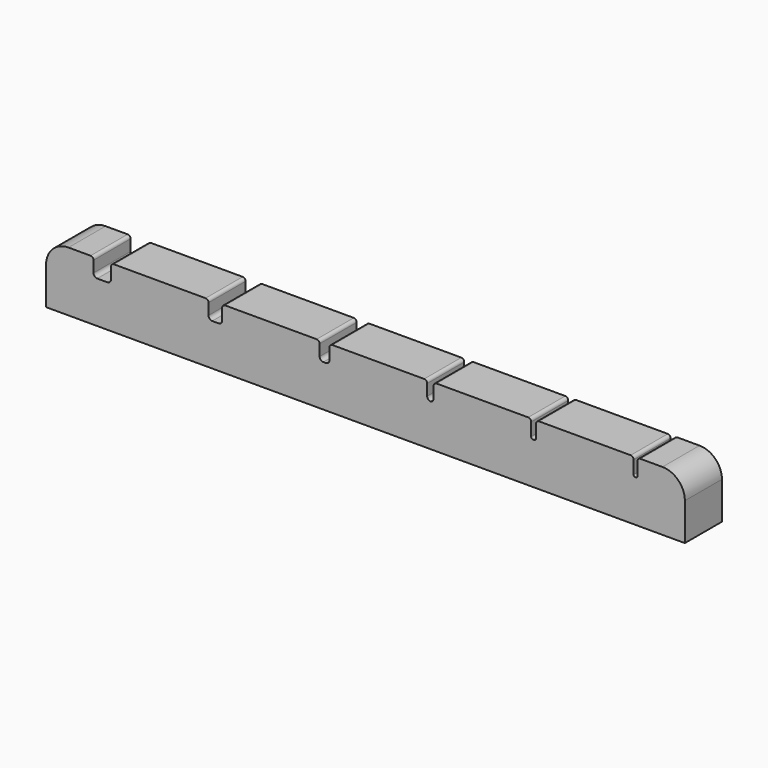
from build123d import *

# Parameters (mm, degrees)
F0_W        = 3.1758
F0_H        = 3.1
F0_W_2      = 1.1684
F0_W_3      = 6.5286
F0_W_4      = 0.9144
F0_W_5      = 6.5226
F0_W_6      = 0.6604
F0_W_7      = 6.5339
F0_W_8      = 0.4318
F0_W_9      = 6.529
F0_W_10     = 0.3302
F0_W_11     = 6.5279
F0_W_12     = 0.254
F0_W_13     = 3.173
F1_DEPTH    = 4
F2_W        = 0.5842
F2_H        = 3.1
F2_W_2      = 0.4572
F2_W_3      = 0.3302
F2_W_4      = 0.2159
F2_W_5      = 0.1651
F2_W_6      = 0.127
F3_DEPTH    = 1.2
F4_T1_DEPTH = 3.1
F5_R        = 0.125
F6_R        = 1.5
F7_R        = 0.2


# Not quite as in the source:
# - a fillet or chamfer that OpenCascade refuses, or shapes differently, is made with other operations: its cross-section is extruded or revolved along the edge and cut away or added


with BuildPart() as f1:
    # F0 (on Top) → F1 (new body)
    with BuildSketch(Plane.XY):
        with Locations((-11.6114438434, -2.5640697926)):
            Rectangle(F0_W, F0_H)
        with Locations((-9.4393438434, -2.5640697926)):
            Rectangle(F0_W_2, F0_H)
        with Locations((-5.5908438434, -2.5640697926)):
            Rectangle(F0_W_3, F0_H)
        with Locations((-1.8693438434, -2.5640697926)):
            Rectangle(F0_W_4, F0_H)
        with Locations((1.8491561566, -2.5640697926)):
            Rectangle(F0_W_5, F0_H)
        with Locations((5.4406561566, -2.5640697926)):
            Rectangle(F0_W_6, F0_H)
        with Locations((9.0378061566, -2.5640697926)):
            Rectangle(F0_W_7, F0_H)
        with Locations((12.5206561566, -2.5640697926)):
            Rectangle(F0_W_8, F0_H)
        with Locations((16.0010561566, -2.5640697926)):
            Rectangle(F0_W_9, F0_H)
        with Locations((19.4306561566, -2.5640697926)):
            Rectangle(F0_W_10, F0_H)
        with Locations((22.8597061566, -2.5640697926)):
            Rectangle(F0_W_11, F0_H)
        with Locations((26.2506561566, -2.5640697926)):
            Rectangle(F0_W_12, F0_H)
        with Locations((27.9641561566, -2.5640697926)):
            Rectangle(F0_W_13, F0_H)
    extrude(amount=F1_DEPTH)

    # F2 (on face) → F3 (cut)
    with BuildSketch(Plane.XY.offset(4)):
        with Locations((-9.1472438434, -2.5640697926)):
            Rectangle(F2_W, F2_H)
        with Locations((-9.7314438434, -2.5640697926)):
            Rectangle(F2_W, F2_H)
        with Locations((-1.6407438434, -2.5640697926)):
            Rectangle(F2_W_2, F2_H)
        with Locations((-2.0979438434, -2.5640697926)):
            Rectangle(F2_W_2, F2_H)
        with Locations((5.2755561566, -2.5640697926)):
            Rectangle(F2_W_3, F2_H)
        with Locations((5.6057561566, -2.5640697926)):
            Rectangle(F2_W_3, F2_H)
        with Locations((12.4127061566, -2.5640697926)):
            Rectangle(F2_W_4, F2_H)
        with Locations((12.6286061566, -2.5640697926)):
            Rectangle(F2_W_4, F2_H)
        with Locations((19.3481061566, -2.5640697926)):
            Rectangle(F2_W_5, F2_H)
        with Locations((19.5132061566, -2.5640697926)):
            Rectangle(F2_W_5, F2_H)
        with Locations((26.3141561566, -2.5640697926)):
            Rectangle(F2_W_6, F2_H)
        with Locations((26.1871561566, -2.5640697926)):
            Rectangle(F2_W_6, F2_H)
    extrude(amount=-F3_DEPTH, mode=Mode.SUBTRACT)

    # F4: fillet of radius 0.25 on 8 edges, made by hand

    # F4_s2 → F4_t1 (join)
    with BuildSketch(Plane.XZ.offset(1.0140697926)):
        with BuildLine():
            ThreePointArc((-10.0235438434, 3.05), (-9.9503205387, 2.8732233047), (-9.7735438434, 2.8))
            Line((-9.7735438434, 2.8), (-10.0235438434, 2.8))
            Line((-10.0235438434, 2.8), (-10.0235438434, 3.05))
        make_face()
        with BuildLine():
            ThreePointArc((-9.1051438434, 2.8), (-8.9283671481, 2.8732233047), (-8.8551438434, 3.05))
            Line((-8.8551438434, 3.05), (-8.8551438434, 2.8))
            Line((-8.8551438434, 2.8), (-9.1051438434, 2.8))
        make_face()
        with BuildLine():
            ThreePointArc((-1.6621438434, 2.8), (-1.4853671481, 2.8732233047), (-1.4121438434, 3.05))
            Line((-1.4121438434, 3.05), (-1.4121438434, 2.8))
            Line((-1.4121438434, 2.8), (-1.6621438434, 2.8))
        make_face()
        with BuildLine():
            ThreePointArc((-2.3265438434, 3.05), (-2.2533205387, 2.8732233047), (-2.0765438434, 2.8))
            Line((-2.0765438434, 2.8), (-2.3265438434, 2.8))
            Line((-2.3265438434, 2.8), (-2.3265438434, 3.05))
        make_face()
        with BuildLine():
            ThreePointArc((5.1104561566, 3.05), (5.1836794613, 2.8732233047), (5.3604561566, 2.8))
            Line((5.3604561566, 2.8), (5.1104561566, 2.8))
            Line((5.1104561566, 2.8), (5.1104561566, 3.05))
        make_face()
        with BuildLine():
            ThreePointArc((5.5208561566, 2.8), (5.6976328519, 2.8732233047), (5.7708561566, 3.05))
            Line((5.7708561566, 3.05), (5.7708561566, 2.8))
            Line((5.7708561566, 2.8), (5.5208561566, 2.8))
        make_face()
        with BuildLine():
            ThreePointArc((12.4865561566, 2.8), (12.6633328519, 2.8732233047), (12.7365561566, 3.05))
            Line((12.7365561566, 3.05), (12.7365561566, 2.8))
            Line((12.7365561566, 2.8), (12.4865561566, 2.8))
        make_face()
        with BuildLine():
            ThreePointArc((12.3047561566, 3.05), (12.3779794613, 2.8732233047), (12.5547561566, 2.8))
            Line((12.5547561566, 2.8), (12.3047561566, 2.8))
            Line((12.3047561566, 2.8), (12.3047561566, 3.05))
        make_face()
    extrude(amount=F4_T1_DEPTH)

    # F5
    f5_edges = [f1.edges().sort_by_distance(p)[0] for p in [
        (19.265556, -2.56407, 2.8),
        (19.595756, -2.56407, 2.8),
        (26.377656, -2.56407, 2.8),
        (26.123656, -2.56407, 2.8),
    ]]
    fillet(f5_edges, radius=F5_R)

    # F6
    f6_edges = [f1.edges().sort_by_distance(p)[0] for p in [
        (29.550656, -2.56407, 4),
        (-13.199344, -2.56407, 4),
    ]]
    fillet(f6_edges, radius=F6_R)

    # F7
    f7_edges = [f1.edges().sort_by_distance(p)[0] for p in [
        (-10.023544, -2.56407, 4),
        (-8.855144, -2.56407, 4),
        (-2.326544, -2.56407, 4),
        (-1.412144, -2.56407, 4),
        (5.110456, -2.56407, 4),
        (5.770856, -2.56407, 4),
        (12.304756, -2.56407, 4),
        (12.736556, -2.56407, 4),
        (19.265556, -2.56407, 4),
        (19.595756, -2.56407, 4),
        (26.123656, -2.56407, 4),
        (26.377656, -2.56407, 4),
    ]]
    fillet(f7_edges, radius=F7_R)


solid = f1.part
